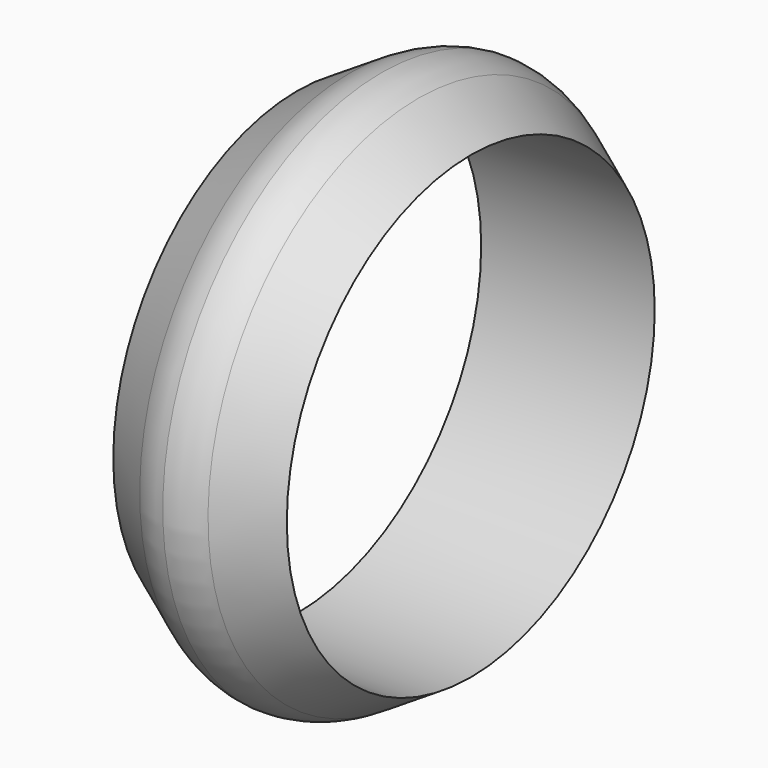
from build123d import *


# Not quite as in the source:
# - a fillet or chamfer that OpenCascade refuses, or shapes differently, is made with other operations: its cross-section is extruded or revolved along the edge and cut away or added
# - a feature of the source that left no trace in its solid (it failed there, or was rolled back) is left out


with BuildPart() as f2:
    # F0 (on Front) → F2 (revolve)
    with BuildSketch(Plane.XZ):
        Polygon((1.27, 20.0025), (0, 20.0025), (-1.27, 20.0025), (-6.35, 16.8275), (6.35, 16.8275), align=None)
    revolve(axis=Axis((4.5157689601, 0, 0), (1, 0, 0)))

    # F4: fillet of radius 5.08 on 2 edges, made by hand

    # F4_s1 → F4_t2 (revolve, cut)
    with BuildSketch(Plane.XZ):
        with BuildLine():
            ThreePointArc((-0.1869248302, 20.0025), (1.2135423361, 19.8056436305), (2.505469785, 19.2303313843))
            Line((2.505469785, 19.2303313843), (1.27, 20.0025))
            Line((1.27, 20.0025), (-0.1869248302, 20.0025))
        make_face()
    revolve(axis=Axis((1.27, 0, 0), (1, 0, 0)), mode=Mode.SUBTRACT)

    # F4_s3 → F4_t4 (revolve, cut)
    with BuildSketch(Plane.XZ):
        with BuildLine():
            ThreePointArc((-0.1869248302, 20.0025), (-1.3792516549, 19.7625268782), (-2.4803658213, 19.2460213617))
            Line((-2.4803658213, 19.2460213617), (-1.27, 20.0025))
            Line((-1.27, 20.0025), (-0.1869248302, 20.0025))
        make_face()
    revolve(axis=Axis((-1.27, 0, 0), (1, 0, 0)), mode=Mode.SUBTRACT)


solid = f2.part
